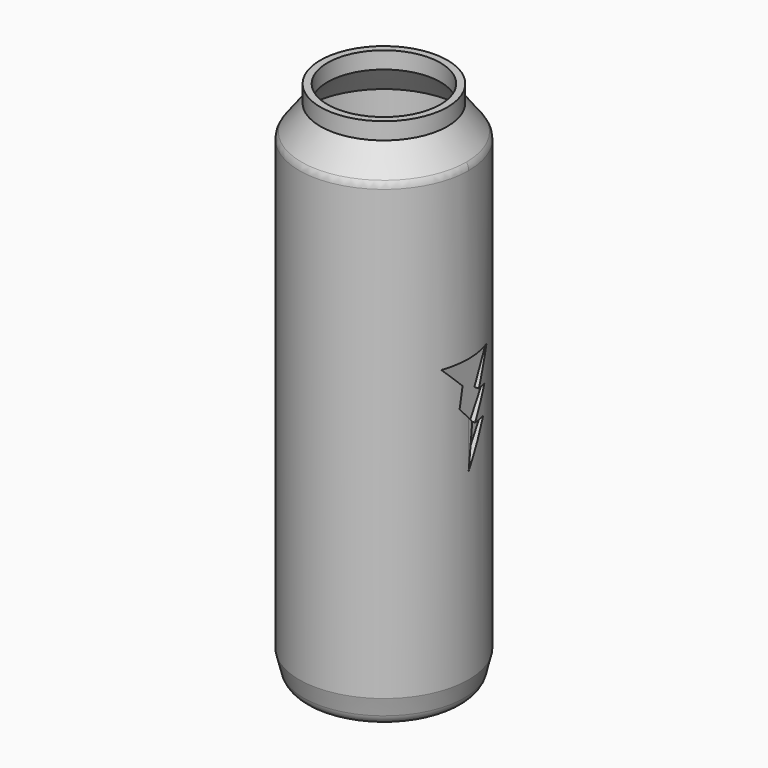
from build123d import *
from build123d import SkipClean  # not in build123d's __all__

# Parameters (mm, degrees)
F0_R      = 38.1
F0_R_2    = 34.925
F1_DEPTH  = 203.2
F3_R      = 34.925
F7_DEPTH  = 2.54
F9_R      = 28.575
F13_DEPTH = 7.62
F10_R     = 25.4
F14_DEPTH = 25.4
F15_R     = 6.35
F16_R     = 5.08
F19_DEPTH = 2.54


with BuildPart() as f1:
    # F0 (on Top) → F1 (new body)
    with BuildSketch(Plane.XY):
        Circle(F0_R)
        Circle(F0_R_2, mode=Mode.SUBTRACT)
    extrude(amount=F1_DEPTH)

    # F4 (on Front) → F6 (revolve)
    with BuildSketch(Plane.XZ):
        Polygon((-38.1, 0), (-34.925, -12.7), (-34.925, 0), align=None)
    revolve(axis=Axis((0, 0, -6.35), (0, 0, -1)))

    # F3 (on offset) → F7 (join)
    with BuildSketch(Plane.XY.offset(-12.7)):
        Circle(F3_R)
    extrude(amount=F7_DEPTH)

    # F11 (on Front) → F12 (revolve)
    with BuildSketch(Plane.XZ):
        Polygon((-25.4, 215.9), (-28.575, 215.9), (-38.1, 203.2), (-34.925, 203.2), align=None)
    revolve(axis=Axis((0, 0, 209.55), (0, 0, -1)))

    # F9 (on offset) → F13 (join)
    with BuildSketch(Plane.XY.offset(215.9)):
        Circle(F9_R)
    extrude(amount=F13_DEPTH)

    # F10 (on offset) → F14 (cut)
    with BuildSketch(Plane.XY.offset(215.9)):
        Circle(F10_R)
    extrude(amount=F14_DEPTH, mode=Mode.SUBTRACT)

    # F15
    f15_edges = [f1.edges().sort_by_distance(p)[0] for p in [
        (34.925, 0, -12.7),
    ]]
    fillet(f15_edges, radius=F15_R)

    # F16
    f16_edges = [f1.edges().sort_by_distance(p)[0] for p in [
        (0, -38.1, 203.2),
        (0, 38.1, 203.2),
    ]]
    fillet(f16_edges, radius=F16_R)

    # F18 (on offset) → F19 (cut)
    with BuildSketch(Plane.YZ.offset(38.1)):
        Polygon((0, 127), (-12.7, 127), (-3.2499410816, 117.5278012156), (-4.7398322865, 108.8000346422), (2.0743066773, 101.2560684681), (0, 82.55), (9.75460466, 100.0966164947), (3.8371453993, 100.0966164947), (10.7981534675, 112.4366257071), (6.3976268284, 112.4366257071), (12.7, 127), align=None)
    with SkipClean():  # cleaning this boolean's faces spoils the solid; the shape is the same uncleaned
        extrude(amount=-F19_DEPTH, mode=Mode.SUBTRACT)


solid = f1.part
